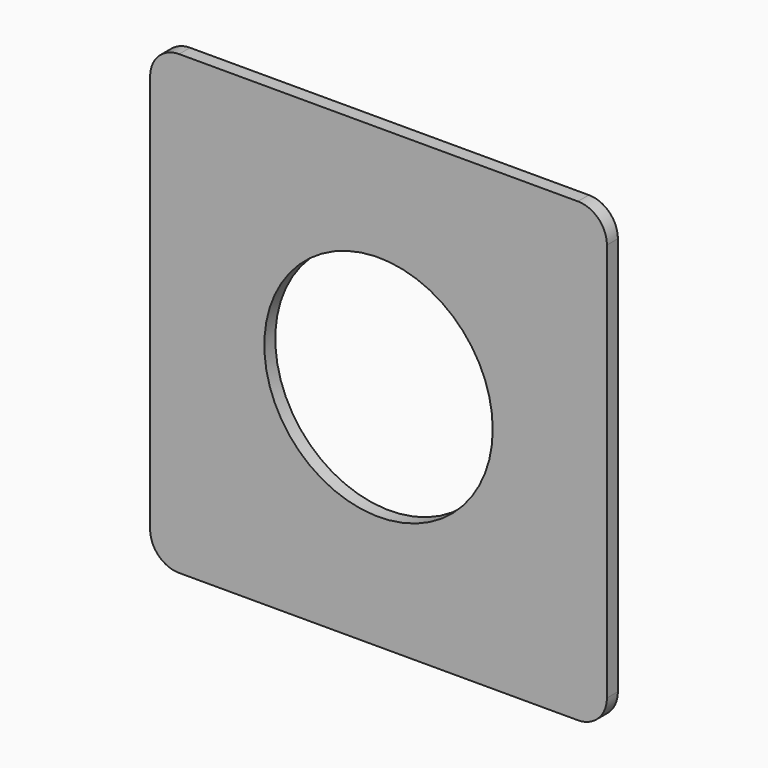
from build123d import *

# Parameters (mm, degrees)
F0_R     = 25
F1_DEPTH = 3


# Not quite as in the source:
# - a feature of the source that left no trace in its solid (it failed there, or was rolled back) is left out


with BuildPart() as f1:
    # F0 (on Front) → F1 (new body)
    with BuildSketch(Plane.XZ):
        with BuildLine():
            Line((43.65, 50), (-43.65, 50))
            ThreePointArc((-43.65, 50), (-48.1401280605, 48.1401280605), (-50, 43.65))
            Line((-50, 43.65), (-50, -43.65))
            ThreePointArc((-50, -43.65), (-48.1401280605, -48.1401280605), (-43.65, -50))
            Line((-43.65, -50), (43.65, -50))
            ThreePointArc((43.65, -50), (48.1401280605, -48.1401280605), (50, -43.65))
            Line((50, -43.65), (50, 43.65))
            ThreePointArc((50, 43.65), (48.1401280605, 48.1401280605), (43.65, 50))
        make_face()
        Circle(F0_R, mode=Mode.SUBTRACT)
    extrude(amount=F1_DEPTH)


solid = f1.part
